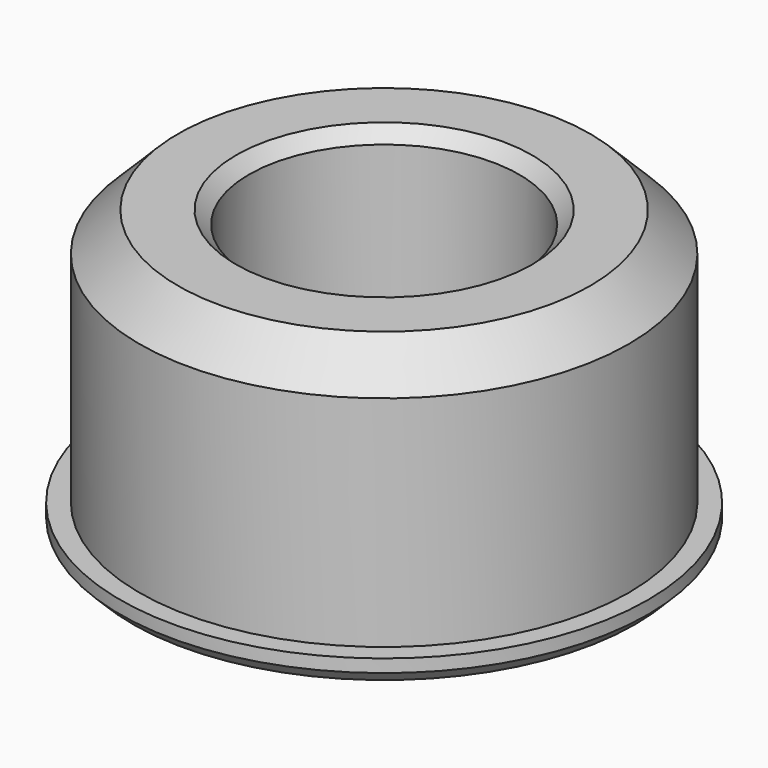
from build123d import *

# Parameters (mm, degrees)
F0_R     = 20.5
F1_DEPTH = 2
F2_R     = 19
F3_DEPTH = 20
F4_D     = 21
F5_SIZE  = 1
F6_SIZE  = 3


with BuildPart() as f1:
    # F0 (on Top) → F1 (new body)
    with BuildSketch(Plane.XY):
        Circle(F0_R)
    extrude(amount=F1_DEPTH)

    # F2 (on face) → F3 (join)
    with BuildSketch(Plane.XY.offset(2)):
        Circle(F2_R)
    extrude(amount=F3_DEPTH)

    # F4 (through all)
    with Locations(Plane(origin=(0, 0, 0), x_dir=(1, 0, 0), z_dir=(0, 0, -1))):
        with Locations((0, 0)):
            Hole(F4_D / 2)

    # F5
    f5_edges = [f1.edges().sort_by_distance(p)[0] for p in [
        (-20.5, 0, 0),
        (-10.5, 0, 0),
        (-10.5, 0, 22),
    ]]
    chamfer(f5_edges, length=F5_SIZE)

    # F6
    f6_edges = [f1.edges().sort_by_distance(p)[0] for p in [
        (-19, 0, 22),
    ]]
    chamfer(f6_edges, length=F6_SIZE)


solid = f1.part
